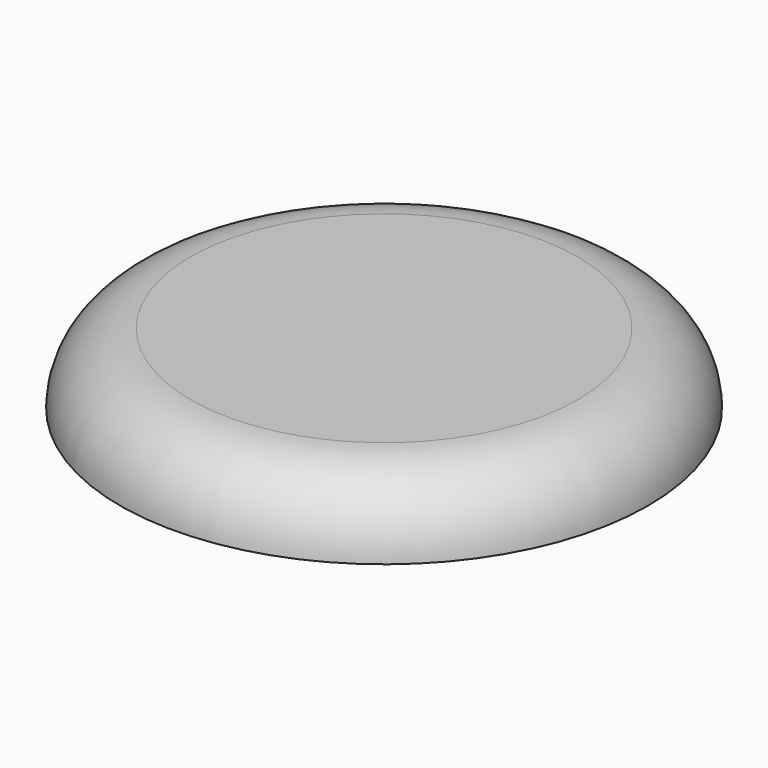
from build123d import *

# Parameters (mm, degrees)
F0_R     = 38.1
F1_DEPTH = 10.16
F2_R     = 10.15999


# Not quite as in the source:
# - a fillet or chamfer is up to 0.001 mm smaller than in the source, because OpenCascade refuses the exact size


with BuildPart() as f1:
    # F0 (on Top) → F1 (new body)
    with BuildSketch(Plane.XY):
        with Locations((-21.9576321542, 17.4457896501)):
            Circle(F0_R)
    extrude(amount=F1_DEPTH)

    # F2 (radius 10.16 in the source; OpenCascade refuses exactly that, so slightly less here)
    f2_edges = [f1.edges().sort_by_distance(p)[0] for p in [
        (-60.057632, 17.44579, 10.16),
    ]]
    fillet(f2_edges, radius=F2_R)


solid = f1.part
